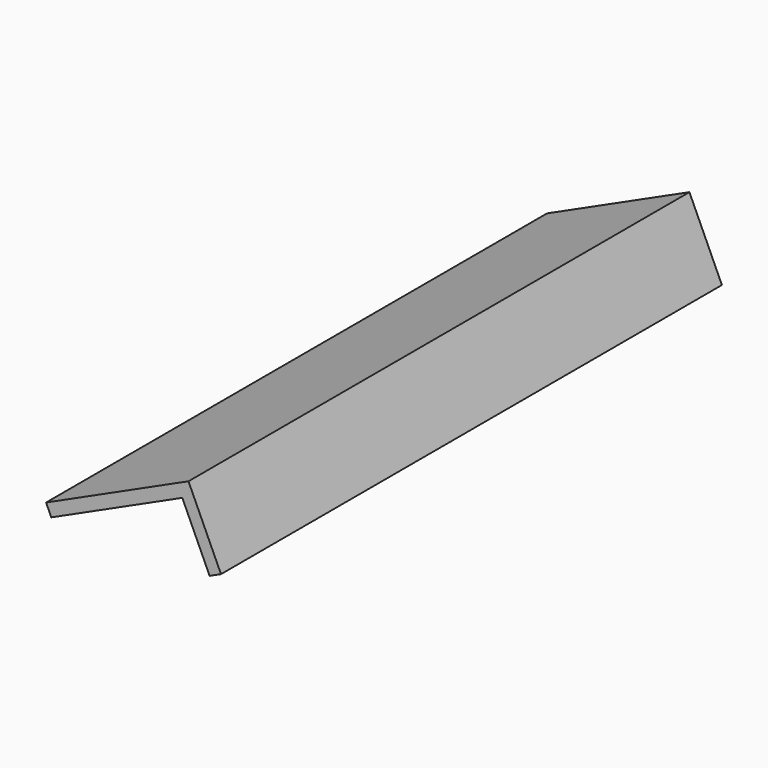
from build123d import *

# Parameters (mm, degrees)
F1_DEPTH = 400


# Not quite as in the source:
# - the program builds the solid bodies; features that only make, move or delete a surface that nothing else refers to are left out


with BuildPart() as f1:
    # F0 (on Front) → F1 (new body)
    with BuildSketch(Plane.XZ):
        Polygon((-90.9688003863, 7.2775040309), (-87.6464615896, 0), (-3.9551652342, 38.2068961622), (13.4871134486, 0), (20.7646174795, 3.3223387967), (0, 48.8067389899), align=None)
    extrude(amount=-F1_DEPTH)


solid = f1.part
